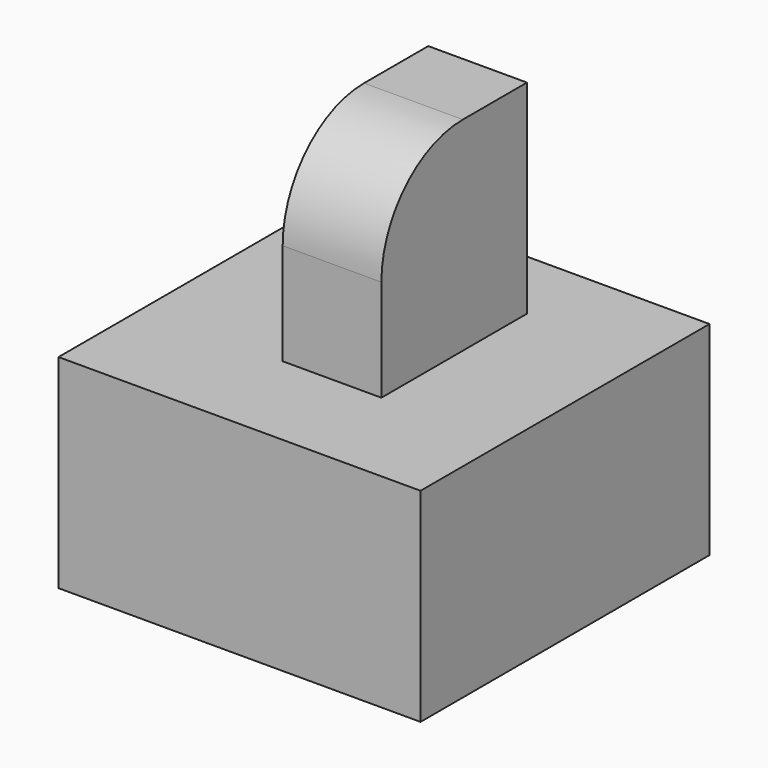
from build123d import *

# Parameters (mm, degrees)
F0_W     = 45.1892055571
F0_H     = 45.0811590999
F1_DEPTH = 25.4
F2_W     = 12.3209874146
F2_H     = 22.7134097368
F3_DEPTH = 25.4
F4_R     = 12.7


# Not quite as in the source:
# - the program builds the solid bodies; features that only make, move or delete a surface that nothing else refers to are left out


with BuildPart() as f1:
    # F0 (on Top) → F1 (new body)
    with BuildSketch(Plane.XY):
        with Locations((0.0014137477, -4.4078445062)):
            Rectangle(F0_W, F0_H)
    extrude(amount=F1_DEPTH)

    # F2 (on face) → F3 (join)
    with BuildSketch(Plane.XY.offset(25.4)):
        with Locations((1.1841731612, -2.6384368539)):
            Rectangle(F2_W, F2_H)
    extrude(amount=F3_DEPTH)

    # F4
    f4_edges = [f1.edges().sort_by_distance(p)[0] for p in [
        (1.184173, -13.995142, 50.8),
    ]]
    fillet(f4_edges, radius=F4_R)


solid = f1.part
